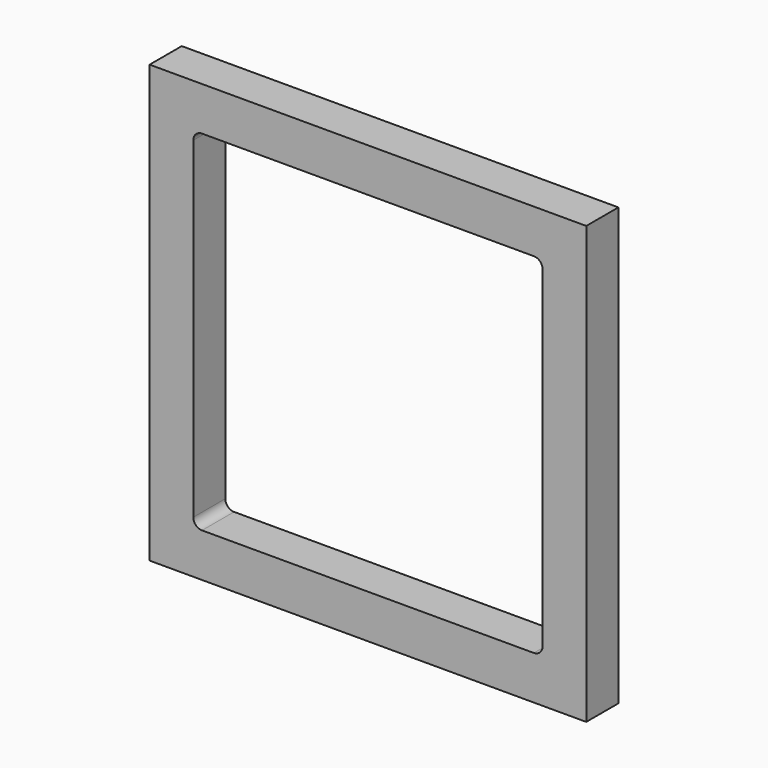
from build123d import *

# Parameters (mm, degrees)
F0_W         = 12700
F0_H         = 12700
F1_DEPTH     = 1168.4
F2_T1_DEPTH  = 9652
F2_T3_DEPTH  = 9652
F2_T6_ANGLE  = 90
F2_T8_ANGLE  = 90
F2_T10_ANGLE = 90
F2_T12_ANGLE = 90


# Not quite as in the source:
# - a fillet or chamfer that OpenCascade refuses, or shapes differently, is made with other operations: its cross-section is extruded or revolved along the edge and cut away or added


with BuildPart() as f1:
    # F0 (on Front) → F1 (new body)
    with BuildSketch(Plane.XZ):
        Rectangle(F0_W, F0_H)
        with BuildLine():
            Line((-5080, -4826), (-5080, 4826))
            ThreePointArc((-5080, 4826), (-5005.6051224214, 5005.6051224214), (-4826, 5080))
            Line((-4826, 5080), (4826, 5080))
            ThreePointArc((4826, 5080), (5005.6051224214, 5005.6051224214), (5080, 4826))
            Line((5080, 4826), (5080, -4826))
            ThreePointArc((5080, -4826), (5005.6051224214, -5005.6051224214), (4826, -5080))
            Line((4826, -5080), (-4826, -5080))
            ThreePointArc((-4826, -5080), (-5005.6051224214, -5005.6051224214), (-5080, -4826))
        make_face(mode=Mode.SUBTRACT)
    extrude(amount=F1_DEPTH)

    # F2: fillet of radius 5.08 on 4 edges, made by hand

    # F2_s2 → F2_t1 (cut)
    with BuildSketch(Plane.YZ.offset(-4826)):
        with BuildLine():
            add(Edge.make_bspline(
                [(-5.08, -5080), (0, -5080), (0, -5085.08)],
                knots=[0, 0, 0, 1, 1, 1], degree=2, weights=[1, 1, 1]))
            Line((0, -5085.08), (0, -5080))
            Line((0, -5080), (-5.08, -5080))
        make_face()
        with BuildLine():
            add(Edge.make_bspline(
                [(-5.08, 5080), (0, 5080), (0, 5085.08)],
                knots=[0, 0, 0, 1, 1, 1], degree=2, weights=[1, 1, 1]))
            Line((0, 5085.08), (0, 5080))
            Line((0, 5080), (-5.08, 5080))
        make_face()
    extrude(amount=F2_T1_DEPTH, mode=Mode.SUBTRACT)

    # F2_s4 → F2_t3 (cut)
    with BuildSketch(Plane.XY.offset(-4826)):
        with BuildLine():
            add(Edge.make_bspline(
                [(-5080, -5.08), (-5080, 0), (-5085.08, 0)],
                knots=[0, 0, 0, 1, 1, 1], degree=2, weights=[1, 1, 1]))
            Line((-5085.08, 0), (-5080, 0))
            Line((-5080, 0), (-5080, -5.08))
        make_face()
        with BuildLine():
            add(Edge.make_bspline(
                [(5080, -5.08), (5080, 0), (5085.08, 0)],
                knots=[0, 0, 0, 1, 1, 1], degree=2, weights=[1, 1, 1]))
            Line((5085.08, 0), (5080, 0))
            Line((5080, 0), (5080, -5.08))
        make_face()
    extrude(amount=F2_T3_DEPTH, mode=Mode.SUBTRACT)

    # F2_s5 → F2_t6 (revolve, cut)
    with BuildSketch(Plane.XY.offset(4826)):
        with BuildLine():
            add(Edge.make_bspline(
                [(-5080, -5.08), (-5080, 0), (-5085.08, 0)],
                knots=[0, 0, 0, 1, 1, 1], degree=2, weights=[1, 1, 1]))
            Line((-5085.08, 0), (-5080, 0))
            Line((-5080, 0), (-5080, -5.08))
        make_face()
    revolve(axis=Axis((-4826, 0, 4826), (0, 1, 0)), revolution_arc=F2_T6_ANGLE, mode=Mode.SUBTRACT)

    # F2_s7 → F2_t8 (revolve, cut)
    with BuildSketch(Plane.YZ.offset(4826)):
        with BuildLine():
            add(Edge.make_bspline(
                [(-5.08, 5080), (0, 5080), (0, 5085.08)],
                knots=[0, 0, 0, 1, 1, 1], degree=2, weights=[1, 1, 1]))
            Line((0, 5085.08), (0, 5080))
            Line((0, 5080), (-5.08, 5080))
        make_face()
    revolve(axis=Axis((4826, 0, 4826), (0, 1, 0)), revolution_arc=F2_T8_ANGLE, mode=Mode.SUBTRACT)

    # F2_s9 → F2_t10 (revolve, cut)
    with BuildSketch(Plane.XY.offset(-4826)):
        with BuildLine():
            add(Edge.make_bspline(
                [(5080, -5.08), (5080, 0), (5085.08, 0)],
                knots=[0, 0, 0, 1, 1, 1], degree=2, weights=[1, 1, 1]))
            Line((5085.08, 0), (5080, 0))
            Line((5080, 0), (5080, -5.08))
        make_face()
    revolve(axis=Axis((4826, 0, -4826), (0, 1, 0)), revolution_arc=F2_T10_ANGLE, mode=Mode.SUBTRACT)

    # F2_s11 → F2_t12 (revolve, cut)
    with BuildSketch(Plane.YZ.offset(-4826)):
        with BuildLine():
            add(Edge.make_bspline(
                [(-5.08, -5080), (0, -5080), (0, -5085.08)],
                knots=[0, 0, 0, 1, 1, 1], degree=2, weights=[1, 1, 1]))
            Line((0, -5085.08), (0, -5080))
            Line((0, -5080), (-5.08, -5080))
        make_face()
    revolve(axis=Axis((-4826, 0, -4826), (0, 1, 0)), revolution_arc=F2_T12_ANGLE, mode=Mode.SUBTRACT)


solid = f1.part
